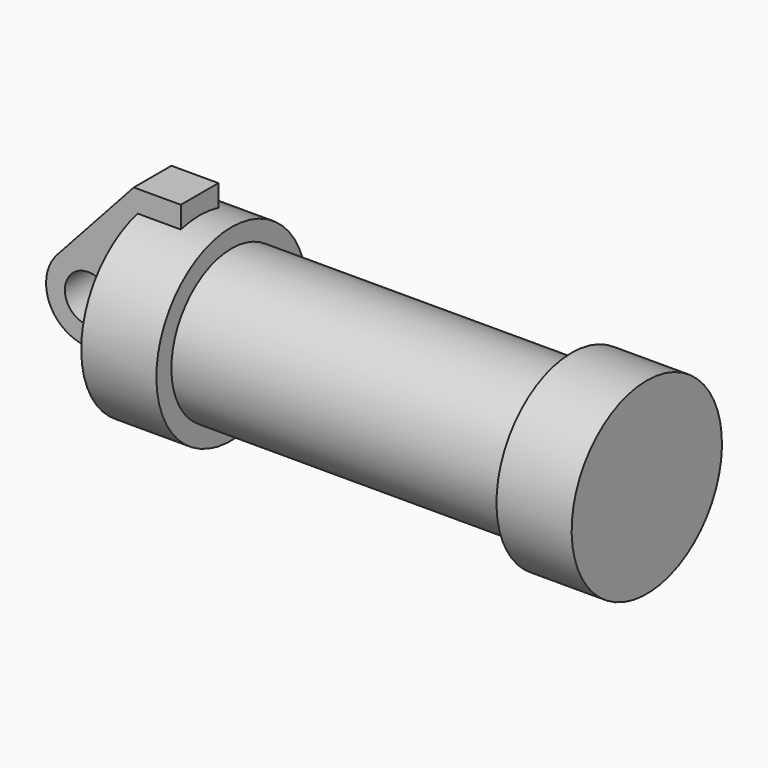
from build123d import *

# Parameters (mm, degrees)
F0_W     = 5.842
F0_H     = 12.7
F0_R     = 3.175
F1_DEPTH = 3.175
F2_DEPTH = 3.175


# Not quite as in the source:
# - the program builds the solid bodies; features that only make, move or delete a surface that nothing else refers to are left out


with BuildPart() as f1:
    # F0 (on Front) → F1 (new body)
    with BuildSketch(Plane.XZ):
        with Locations((2.921, 6.35)):
            Rectangle(F0_W, F0_H)
        with BuildLine():
            Line((-0.9398, 0), (0, 0))
            Line((0, 0), (0, 12.7))
            Line((0, 12.7), (5.842, 12.7))
            Line((5.842, 12.7), (5.842, 15.24))
            Line((5.842, 15.24), (-0.508, 15.24))
            Line((-0.508, 15.24), (-10.8806298187, 3.8475430269))
            ThreePointArc((-10.8806298187, 3.8475430269), (-4.5919612295, 5.3297205562), (-0.9398, 0))
        make_face()
        with BuildLine():
            Line((5.842, 0), (0, 0))
            Line((0, 0), (-0.9398, 0))
            ThreePointArc((-0.9398, 0), (-3.1957909266, -4.5493385486), (-8.1826630726, -5.5069827884))
            Line((-8.1826630726, -5.5069827884), (5.842, -9.398))
            Line((5.842, -9.398), (5.842, 0))
        make_face()
        with BuildLine():
            ThreePointArc((-8.1826630726, -5.5069827884), (-3.1957909266, -4.5493385486), (-0.9398, 0))
            ThreePointArc((-0.9398, 0), (-4.5919612295, 5.3297205562), (-10.8806298187, 3.8475430269))
            ThreePointArc((-10.8806298187, 3.8475430269), (-12.1459778134, -1.5837270034), (-8.1826630726, -5.5069827884))
        make_face()
        with Locations((-6.6548, 0)):
            Circle(F0_R, mode=Mode.SUBTRACT)
    extrude(amount=-F1_DEPTH)

    # F0 (on Front) → F2 (join)
    with BuildSketch(Plane.XZ):
        with BuildLine():
            Line((5.842, 0), (0, 0))
            Line((0, 0), (-0.9398, 0))
            ThreePointArc((-0.9398, 0), (-3.1957909266, -4.5493385486), (-8.1826630726, -5.5069827884))
            Line((-8.1826630726, -5.5069827884), (5.842, -9.398))
            Line((5.842, -9.398), (5.842, 0))
        make_face()
        with Locations((2.921, 6.35)):
            Rectangle(F0_W, F0_H)
        with BuildLine():
            Line((-0.9398, 0), (0, 0))
            Line((0, 0), (0, 12.7))
            Line((0, 12.7), (5.842, 12.7))
            Line((5.842, 12.7), (5.842, 15.24))
            Line((5.842, 15.24), (-0.508, 15.24))
            Line((-0.508, 15.24), (-10.8806298187, 3.8475430269))
            ThreePointArc((-10.8806298187, 3.8475430269), (-4.5919612295, 5.3297205562), (-0.9398, 0))
        make_face()
        with BuildLine():
            ThreePointArc((-8.1826630726, -5.5069827884), (-3.1957909266, -4.5493385486), (-0.9398, 0))
            ThreePointArc((-0.9398, 0), (-4.5919612295, 5.3297205562), (-10.8806298187, 3.8475430269))
            ThreePointArc((-10.8806298187, 3.8475430269), (-12.1459778134, -1.5837270034), (-8.1826630726, -5.5069827884))
        make_face()
        with Locations((-6.6548, 0)):
            Circle(F0_R, mode=Mode.SUBTRACT)
    extrude(amount=F2_DEPTH)


with BuildPart() as f3:
    # F0 (on Front) → F3 (revolve)
    with BuildSketch(Plane.XZ):
        with Locations((2.921, 6.35)):
            Rectangle(F0_W, F0_H)
        Polygon((5.842, 12.7), (5.842, 0), (66.294, 0), (66.294, 12.7), (56.134, 12.7), (56.134, 10.16), (10.16, 10.16), (10.16, 12.7), align=None)
    revolve(axis=Axis((33.147, 0, 0), (-1, 0, 0)))


solid = Compound([f1.part, f3.part])
